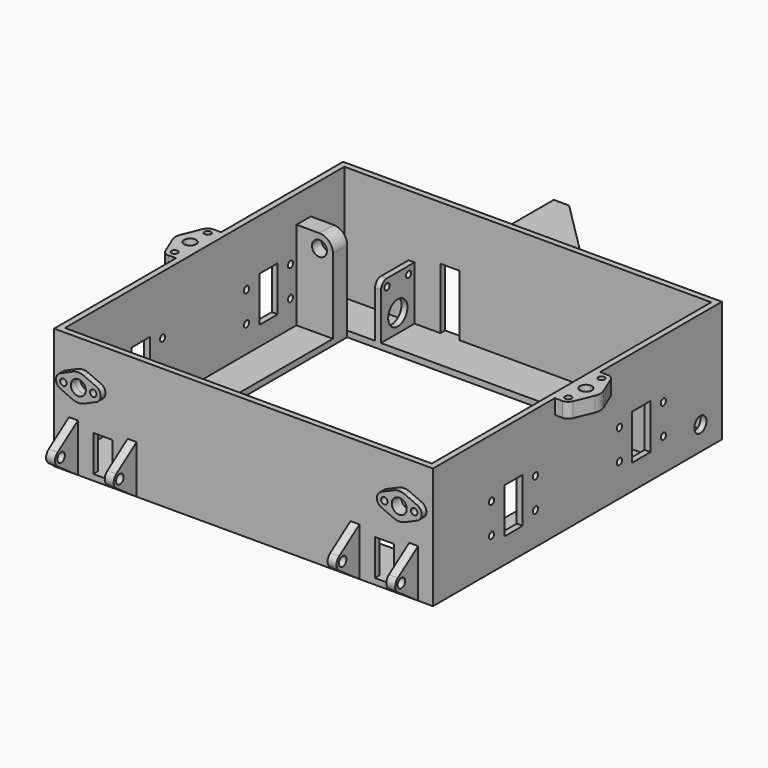
from build123d import *

# Parameters (mm, degrees)
F0_W      = 201.952733
F0_H      = 192.556511
F0_W_2    = 156.7277282
F0_H_2    = 141.5065242
F1_DEPTH  = 3.175
F2_W      = 201.952733
F2_H      = 192.556511
F2_W_2    = 195.602733
F2_H_2    = 186.206511
F3_DEPTH  = 61.4624374
F4_W      = 19.4375024
F4_H      = 9.525
F5_DEPTH  = 47.2163394
F6_R      = 4
F7_DEPTH  = 6.35
F8_R      = 7.1750047
F9_W      = 3.175
F9_H      = 22.3499934
F10_DEPTH = 28.7625282
F11_R     = 6.4124967
F11_R_2   = 1.7272
F12_DEPTH = 127
F13_R     = 3.96875
F14_R     = 4.087495
F15_DEPTH = 201.952733
F17_DEPTH = 46.1809846
F18_SIZE  = 43.0059846
F19_R     = 11.2530001
F19_R_2   = 1.5
F20_DEPTH = 5
F21_W     = 10.1750114
F21_H     = 32.6154923
F22_DEPTH = 189.381511
F23_W     = 30.0434756
F23_H     = 7.9375
F24_DEPTH = 50.8
F25_W     = 4.7625
F25_H     = 25.6500376
F26_DEPTH = 25.4
F27_R     = 2.5
F28_DEPTH = 186.1277456
F29_W     = 10.1750114
F29_H     = 19.3000376
F30_DEPTH = 3.175
F31_W     = 30.0434756
F31_H     = 7.9375
F32_DEPTH = 50.8
F33_R     = 1.7272
F33_R_2   = 3.175
F34_DEPTH = 7.9375
F35_W     = 12.2546872
F35_H     = 24
F35_R     = 1.7272
F36_DEPTH = 201.952733
F37_R     = 4
F38_DEPTH = 3.175
F39_R     = 4
F40_DEPTH = 3.175
F41_R     = 1.7272
F42_DEPTH = 6.35


# Not quite as in the source:
# - an extrude ends at something that could not be found from the text; its depth is read off the source's solid


with BuildPart() as f1:
    # F0 (on Top) → F1 (new body)
    with BuildSketch(Plane.XY):
        with Locations((78.3638641, -70.7532621)):
            Rectangle(F0_W, F0_H)
        with Locations((78.3638641, -70.7532621)):
            Rectangle(F0_W_2, F0_H_2, mode=Mode.SUBTRACT)
    extrude(amount=F1_DEPTH)

    # F2 (on face) → F3 (join)
    with BuildSketch(Plane.XY.offset(3.175)):
        with Locations((78.3638641, -70.7532621)):
            Rectangle(F2_W, F2_H)
        with Locations((78.3638641, -70.7532621)):
            Rectangle(F2_W_2, F2_H_2, mode=Mode.SUBTRACT)
    extrude(amount=F3_DEPTH)

    # F4 (on face) → F5 (join)
    with BuildSketch(Plane.XY.offset(3.175)):
        with Locations((-9.7187512, -4.7625)):
            Rectangle(F4_W, F4_H)
        with Locations((166.4464794, -4.7625)):
            Rectangle(F4_W, F4_H)
    extrude(amount=F5_DEPTH)

    # F6 (on face) → F7 (cut)
    with BuildSketch(Plane.XZ.offset(9.525)):
        with Locations((163.9027329, 43.2163347)):
            Circle(F6_R)
        with Locations((-7.1750047, 43.2163347)):
            Circle(F6_R)
    extrude(amount=-F7_DEPTH, mode=Mode.SUBTRACT)

    # F8
    f8_edges = [f1.edges().sort_by_distance(p)[0] for p in [
        (156.727728, -4.7625, 50.391339),
        (0, -4.7625, 50.391339),
    ]]
    fillet(f8_edges, radius=F8_R)

    # F9 (on face) → F10 (join)
    with BuildSketch(Plane.XY.offset(3.175)):
        with Locations((16.4513641, 11.1749967)):
            Rectangle(F9_W, F9_H)
        with Locations((140.2763641, 11.1749967)):
            Rectangle(F9_W, F9_H)
    extrude(amount=F10_DEPTH)

    # F11 (on face) → F12 (cut, through all)
    with BuildSketch(Plane(origin=(14.8638641, 0, 0), x_dir=(0, -1, 0), z_dir=(-1, 0, 0))):
        with Locations((-11.1749967, 12.8250061)):
            Circle(F11_R)
        with Locations((-18.3812434, 27.9687782)):
            Circle(F11_R_2)
        with Locations((-3.96875, 27.9687782)):
            Circle(F11_R_2)
    extrude(amount=-F12_DEPTH, mode=Mode.SUBTRACT)

    # F13
    f13_edges = [f1.edges().sort_by_distance(p)[0] for p in [
        (16.451364, 0, 31.937528),
        (140.276364, 0, 31.937528),
    ]]
    fillet(f13_edges, radius=F13_R)

    # F14 (on face) → F15 (cut, through all)
    with BuildSketch(Plane(origin=(-22.6125024, 0, 0), x_dir=(0, -1, 0), z_dir=(-1, 0, 0))):
        with Locations((-11.1749967001, 12.8250061)):
            Circle(F14_R)
    extrude(amount=-F15_DEPTH, mode=Mode.SUBTRACT)

    # F16 (on face) → F17 (join)
    with BuildSketch(Plane(origin=(0, 25.5249934, 0), x_dir=(-1, 0, 0), z_dir=(0, 1, 0))):
        Polygon((-103.9543564, 3.175), (-103.9543564, 0), (-52.7733718, 0), (-52.7733718, 52.5309846), (-103.9543564, 52.5309846), (-103.9543564, 49.3559846), (-57.7733718, 49.3559846), (-57.7733718, 3.175), align=None)
    extrude(amount=F17_DEPTH)

    # F18
    f18_edges = [f1.edges().sort_by_distance(p)[0] for p in [
        (103.954356, 71.705978, 1.5875),
        (103.954356, 71.705978, 50.943485),
    ]]
    chamfer(f18_edges, length=F18_SIZE)

    # F19 (on face) → F20 (cut, through all)
    with BuildSketch(Plane(origin=(52.7733718, 0, 0), x_dir=(0, -1, 0), z_dir=(-1, 0, 0))):
        with Locations((-50.2029857, 26.2654923)):
            Circle(F19_R)
        with Locations((-34.7029913, 10.7654979)):
            Circle(F19_R_2)
        with Locations((-65.7029801, 10.7654979)):
            Circle(F19_R_2)
        with Locations((-65.7029801, 41.7654867)):
            Circle(F19_R_2)
        with Locations((-34.7029913, 41.7654867)):
            Circle(F19_R_2)
    extrude(amount=-F20_DEPTH, mode=Mode.SUBTRACT)

    # F21 (on face) → F22 (cut, through all)
    with BuildSketch(Plane(origin=(0, 25.5249934, 0), x_dir=(-1, 0, 0), z_dir=(0, 1, 0))):
        with Locations((-36.8608687, 19.48274615)):
            Rectangle(F21_W, F21_H)
    extrude(amount=-F22_DEPTH, mode=Mode.SUBTRACT)

    # F23 (on face) → F24 (join)
    with BuildSketch(Plane(origin=(-22.6125024, 0, 0), x_dir=(0, -1, 0), z_dir=(-1, 0, 0))):
        with Locations((70.7532621, 60.6686874)):
            Rectangle(F23_W, F23_H)
    extrude(amount=F24_DEPTH)

    # F25 (on face) → F26 (join)
    with BuildSketch(Plane.XZ.offset(167.0315176)):
        with Locations((169.0464869, 12.8250188)):
            Rectangle(F25_W, F25_H)
        with Locations((137.7589701, 12.8250188)):
            Rectangle(F25_W, F25_H)
        with Locations((18.9687581, 12.8250188)):
            Rectangle(F25_W, F25_H)
        with Locations((-12.3187587, 12.8250188)):
            Rectangle(F25_W, F25_H)
    extrude(amount=F26_DEPTH)

    # F27 (on face) → F28 (cut, through all)
    with BuildSketch(Plane(origin=(-14.7000087, 0, 0), x_dir=(0, -1, 0), z_dir=(-1, 0, 0))):
        with Locations((178.206527, 12.8250188)):
            Circle(F27_R)
        with BuildLine():
            Line((180.5527256577, 9.4779354079), (167.0315176, 0))
            Line((167.0315176, 0), (192.4315176, 0))
            Line((192.4315176, 0), (192.4315176, 25.6500376))
            Line((192.4315176, 25.6500376), (167.0315176, 25.6500376))
            Line((167.0315176, 25.6500376), (180.5527256577, 16.1721021921))
            ThreePointArc((180.5527256577, 16.1721021921), (182.294022, 12.8250188), (180.5527256577, 9.4779354079))
        make_face()
    extrude(amount=-F28_DEPTH, mode=Mode.SUBTRACT)

    # F29 (on face) → F30 (cut, through all)
    with BuildSketch(Plane.XZ.offset(167.0315176)):
        with Locations((153.4027285, 12.8250188)):
            Rectangle(F29_W, F29_H)
        with Locations((3.3249997, 12.8250188)):
            Rectangle(F29_W, F29_H)
    extrude(amount=-F30_DEPTH, mode=Mode.SUBTRACT)

    # F31 (on face) → F32 (join)
    with BuildSketch(Plane.YZ.offset(179.3402306)):
        with Locations((-70.7532621, 60.6686874)):
            Rectangle(F31_W, F31_H)
    extrude(amount=F32_DEPTH)

    # F33 (on face) → F34 (cut, through all)
    with BuildSketch(Plane(origin=(0, 0, 56.6999374), x_dir=(1, 0, 0), z_dir=(0, 0, -1))):
        with BuildLine():
            ThreePointArc((-30.2468781415, 83.3274877137), (-28.7850631892, 85.1068853794), (-26.5812524, 85.7749999))
            Line((-26.5812524, 85.7749999), (-73.4125024, 85.7749999))
            Line((-73.4125024, 85.7749999), (-73.4125024, 55.7315243))
            Line((-73.4125024, 55.7315243), (-26.5812524, 55.7315243))
            ThreePointArc((-26.5812524, 55.7315243), (-28.7850631892, 56.3996388206), (-30.2468781415, 58.1790364863))
            Line((-30.2468781415, 58.1790364863), (-34.2410333478, 67.803487054))
            ThreePointArc((-34.2410333478, 67.803487054), (-34.8288102, 70.7532621), (-34.2410333478, 73.703037146))
            Line((-34.2410333478, 73.703037146), (-30.2468781415, 83.3274877137))
        make_face()
        with Locations((-26.5812524, 81.8062499)):
            Circle(F33_R)
        with Locations((-27.1331563, 70.7532621)):
            Circle(F33_R_2)
        with Locations((-26.5812524, 59.7002743)):
            Circle(F33_R)
        with Locations((183.8608845, 70.7532621)):
            Circle(F33_R_2)
        with BuildLine():
            Line((230.1402306, 85.7749999), (183.3089806, 85.7749999))
            ThreePointArc((183.3089806, 85.7749999), (185.5127913892, 85.1068853794), (186.9746063415, 83.3274877137))
            Line((186.9746063415, 83.3274877137), (190.9687615478, 73.703037146))
            ThreePointArc((190.9687615478, 73.703037146), (191.5565384, 70.7532621), (190.9687615478, 67.803487054))
            Line((190.9687615478, 67.803487054), (186.9746063415, 58.1790364863))
            ThreePointArc((186.9746063415, 58.1790364863), (185.5127913892, 56.3996388206), (183.3089806, 55.7315243))
            Line((183.3089806, 55.7315243), (230.1402306, 55.7315243))
            Line((230.1402306, 55.7315243), (230.1402306, 85.7749999))
        make_face()
        with Locations((183.3089806, 81.8062499)):
            Circle(F33_R)
        with Locations((183.3089806, 59.7002743)):
            Circle(F33_R)
    extrude(amount=-F34_DEPTH, mode=Mode.SUBTRACT)

    # F35 (on face) → F36 (cut, through all)
    with BuildSketch(Plane.YZ.offset(179.3402306)):
        with Locations((-113.3690265, 25.4)):
            Rectangle(F35_W, F35_H)
        with Locations((-28.1374977, 25.4)):
            Rectangle(F35_W, F35_H)
        with Locations((-128.0127742, 33.4312514)):
            Circle(F35_R)
        with Locations((-128.0127742, 17.3687486)):
            Circle(F35_R)
        with Locations((-98.7252788, 17.3687486)):
            Circle(F35_R)
        with Locations((-98.7252788, 33.4312514)):
            Circle(F35_R)
        with Locations((-42.7812454, 33.4312514)):
            Circle(F35_R)
        with Locations((-42.7812454, 17.3687486)):
            Circle(F35_R)
        with Locations((-13.49375, 17.3687486)):
            Circle(F35_R)
        with Locations((-13.49375, 33.4312514)):
            Circle(F35_R)
    extrude(amount=-F36_DEPTH, mode=Mode.SUBTRACT)

    # F37 (on face) → F38 (cut, through all)
    with BuildSketch(Plane.XZ.offset(167.0315176)):
        with Locations((-7.1750047, 43.2163347)):
            Circle(F37_R)
        with Locations((163.9027329, 43.2163347)):
            Circle(F37_R)
    extrude(amount=-F38_DEPTH, mode=Mode.SUBTRACT)

    # F39 (on face) → F40 (join)
    with BuildSketch(Plane.XZ.offset(167.0315176)):
        with BuildLine():
            Line((166.789604831, 36.6477366263), (173.468317151, 39.5830033172))
            ThreePointArc((173.468317151, 39.5830033172), (175.8402329, 43.2163347), (173.468317151, 46.8496660828))
            Line((173.468317151, 46.8496660828), (166.789604831, 49.7849327737))
            ThreePointArc((166.789604831, 49.7849327737), (163.9027329, 50.3913267), (161.015860969, 49.7849327737))
            Line((161.015860969, 49.7849327737), (154.337148649, 46.8496660828))
            ThreePointArc((154.337148649, 46.8496660828), (151.9652329, 43.2163347), (154.337148649, 39.5830033172))
            Line((154.337148649, 39.5830033172), (161.015860969, 36.6477366263))
            ThreePointArc((161.015860969, 36.6477366263), (163.9027329, 36.0413427), (166.789604831, 36.6477366263))
        make_face()
        with Locations((163.9027329, 43.2163347)):
            Circle(F39_R, mode=Mode.SUBTRACT)
        with BuildLine():
            Line((-10.061876631, 49.7849327737), (-16.740588951, 46.8496660828))
            ThreePointArc((-16.740588951, 46.8496660828), (-19.1125047, 43.2163347), (-16.740588951, 39.5830033172))
            Line((-16.740588951, 39.5830033172), (-10.061876631, 36.6477366263))
            ThreePointArc((-10.061876631, 36.6477366263), (-7.1750047, 36.0413427), (-4.288132769, 36.6477366263))
            Line((-4.288132769, 36.6477366263), (2.390579551, 39.5830033172))
            ThreePointArc((2.390579551, 39.5830033172), (4.7624953, 43.2163347), (2.390579551, 46.8496660828))
            Line((2.390579551, 46.8496660828), (-4.288132769, 49.7849327737))
            ThreePointArc((-4.288132769, 49.7849327737), (-7.1750047, 50.3913267), (-10.061876631, 49.7849327737))
        make_face()
        with Locations((-7.1750047, 43.2163347)):
            Circle(F39_R, mode=Mode.SUBTRACT)
    extrude(amount=F40_DEPTH)

    # F41 (on face) → F42 (cut, through all)
    with BuildSketch(Plane.XZ.offset(170.2065176)):
        with Locations((0.7937453, 43.2163347)):
            Circle(F41_R)
        with Locations((-15.1437547, 43.2163347)):
            Circle(F41_R)
        with Locations((171.8714829, 43.2163347)):
            Circle(F41_R)
        with Locations((155.9339829, 43.2163347)):
            Circle(F41_R)
    extrude(amount=-F42_DEPTH, mode=Mode.SUBTRACT)


solid = f1.part
